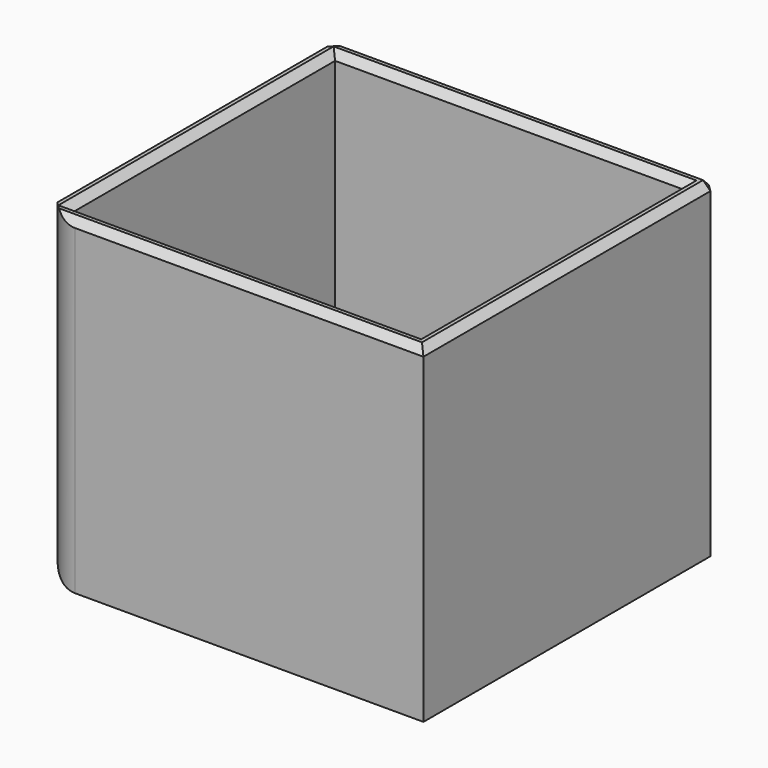
from build123d import *

# Parameters (mm, degrees)
F0_W        = 52.5702424347
F0_H        = 44.9169911444
F1_DEPTH    = 25
F2_DEPTH    = 25
F3_T        = -2.5
F4_SIZE     = 1
F5_T1_DEPTH = 68.9169911444
F5_T3_DEPTH = 6.1776694265
F5_T5_DEPTH = 48.0000001753
F5_T7_DEPTH = 6.1776694575
F5_T9_DEPTH = 75


# Not quite as in the source:
# - a fillet or chamfer that OpenCascade refuses, or shapes differently, is made with other operations: its cross-section is extruded or revolved along the edge and cut away or added


with BuildPart() as f1:
    # F0 (on Front) → F1 (new body)
    with BuildSketch(Plane.XZ):
        with Locations((26.2851212174, 22.4584955722)):
            Rectangle(F0_W, F0_H)
    extrude(amount=F1_DEPTH)

    # F2 (add): a face of the model
    f2_faces = [f1.faces().sort_by_distance(p)[0] for p in [
        (26.2851212174, -25, 22.4584955722),
    ]]
    extrude(f2_faces, amount=F2_DEPTH)

    # F3
    f3_openings = [f1.faces().sort_by_distance(p)[0] for p in [
        (26.285121, -25, 44.916991),
    ]]
    offset(amount=F3_T, openings=f3_openings)

    # F4
    f4_edges = [f1.edges().sort_by_distance(p)[0] for p in [
        (52.570242, 0, 22.458496),
        (52.570242, -25, 44.916991),
        (26.285121, -50, 44.916991),
        (0, -25, 44.916991),
        (26.285121, 0, 44.916991),
        (2.5, -25, 44.916991),
        (26.285121, -47.5, 44.916991),
        (50.070242, -25, 44.916991),
        (26.285121, -2.5, 44.916991),
    ]]
    chamfer(f4_edges, length=F4_SIZE)

    # F5: fillet of radius 5 on 4 edges, made by hand

    # F5_s2 → F5_t1 (cut)
    with BuildSketch(Plane.XY.offset(-12.5)):
        with BuildLine():
            ThreePointArc((0, -45), (1.4644660941, -48.5355339059), (5, -50))
            Line((5, -50), (0, -50))
            Line((0, -50), (0, -45))
        make_face()
        with BuildLine():
            ThreePointArc((0, -5), (1.4644660941, -1.4644660941), (5, 0))
            Line((5, 0), (0, 0))
            Line((0, 0), (0, -5))
        make_face()
    extrude(amount=F5_T1_DEPTH, mode=Mode.SUBTRACT)

    # F5_s4 → F5_t3 (cut)
    with BuildSketch(Plane.XZ.offset(49.0000001032)):
        with BuildLine():
            ThreePointArc((0, 41.8459233326), (0.3806023374, 43.7593404944), (1.4644660941, 45.3814572385))
            Line((1.4644660941, 45.3814572385), (0, 43.9169911444))
            Line((0, 43.9169911444), (0, 41.8459233326))
        make_face()
    extrude(amount=F5_T3_DEPTH, mode=Mode.SUBTRACT)

    # F5_s6 → F5_t5 (cut)
    with BuildSketch(Plane.XZ.offset(0.9999999279)):
        with BuildLine():
            ThreePointArc((0, 41.9169911444), (0.2565835097, 43.4981299745), (1, 44.9169911444))
            Line((1, 44.9169911444), (0, 43.9169911444))
            Line((0, 43.9169911444), (0, 41.9169911444))
        make_face()
    extrude(amount=F5_T5_DEPTH, mode=Mode.SUBTRACT)

    # F5_s8 → F5_t7 (cut)
    with BuildSketch(Plane.XZ.offset(-5.1776695297)):
        with BuildLine():
            ThreePointArc((0, 41.8459233326), (0.3806023374, 43.7593404944), (1.4644660941, 45.3814572385))
            Line((1.4644660941, 45.3814572385), (0, 43.9169911444))
            Line((0, 43.9169911444), (0, 41.8459233326))
        make_face()
    extrude(amount=F5_T7_DEPTH, mode=Mode.SUBTRACT)

    # F5_s10 → F5_t9 (cut)
    with BuildSketch(Plane.XZ.offset(-12.5)):
        with BuildLine():
            ThreePointArc((0, 5), (1.4644660941, 1.4644660941), (5, 0))
            Line((5, 0), (0, 0))
            Line((0, 0), (0, 5))
        make_face()
    extrude(amount=F5_T9_DEPTH, mode=Mode.SUBTRACT)


solid = f1.part
